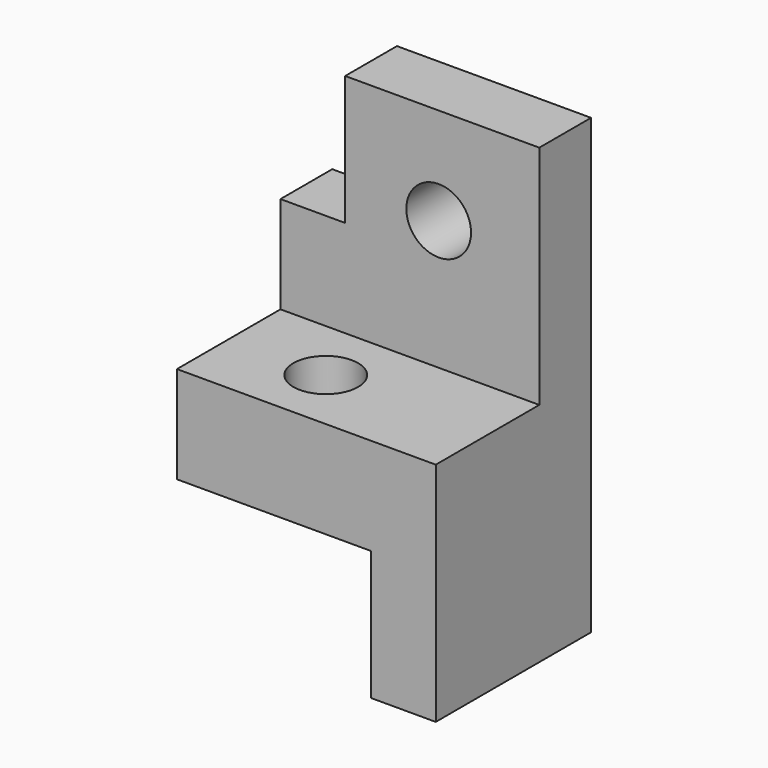
from build123d import *

# Parameters (mm, degrees)
F0_R     = 5
F1_DEPTH = 10
F2_DEPTH = 30
F3_R     = 5
F4_DEPTH = 25


# Not quite as in the source:
# - a feature names something its author has since deleted; it is built from what else it names


with BuildPart() as f1:
    # F0 (on Front) → F1 (new body)
    with BuildSketch(Plane.XZ):
        Polygon((-10.0340604992, 15.3177212924), (-20.0340604992, 15.3177212924), (-20.0340604992, 0.3177212924), (19.9659395008, 0.3177212924), (19.9659395008, 35.3177212924), (-10.0340604992, 35.3177212924), align=None)
        with Locations((4.4167656451, 20.3177212924)):
            Circle(F0_R, mode=Mode.SUBTRACT)
        Polygon((19.9659395008, 0.3177212924), (-20.0340604992, 0.3177212924), (-20.0340604992, -14.6822787076), (9.9659395008, -14.6822787076), (9.9659395008, -34.6822787076), (19.9659395008, -34.6822787076), align=None)
    extrude(amount=F1_DEPTH)

    # F0 (on Front) → F2 (join)
    with BuildSketch(Plane.XZ):
        Polygon((19.9659395008, 0.3177212924), (-20.0340604992, 0.3177212924), (-20.0340604992, -14.6822787076), (9.9659395008, -14.6822787076), (9.9659395008, -34.6822787076), (19.9659395008, -34.6822787076), align=None)
    extrude(amount=F2_DEPTH)

    # F3 (on face) → F4 (cut)
    with BuildSketch(Plane(origin=(0, 0, -14.6822787076), x_dir=(1, 0, 0), z_dir=(0, 0, -1))):
        with Locations((-5.0340604992, 20)):
            Circle(F3_R)
    extrude(amount=-F4_DEPTH, mode=Mode.SUBTRACT)


solid = f1.part
